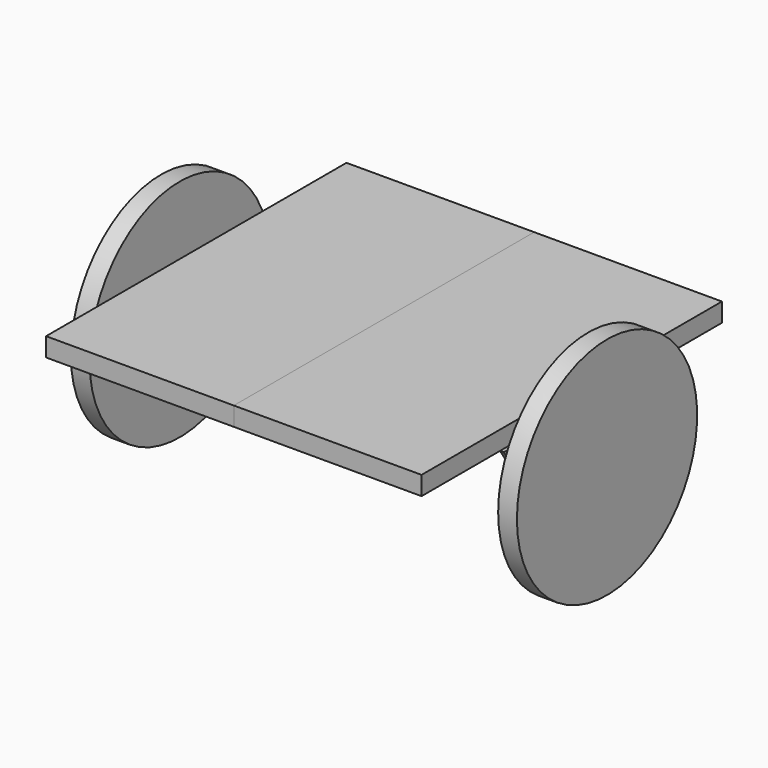
from build123d import *

# Parameters (mm, degrees)
F0_W      = 127
F0_H      = 254
F1_DEPTH  = 12.7
F3_DEPTH  = 11.176
F4_R      = 76.2
F5_DEPTH  = 12.7
F7_DEPTH  = 2.54
F12_R     = 6.556935049
F13_DEPTH = 12.7
F14_W     = 20.32
F14_H     = 45.72
F15_DEPTH = 6.35
F16_W     = 20.32
F16_H     = 22.86
F17_DEPTH = 29.972
F19_START = -3.81
F18_R     = 26.2593452301
F19_DEPTH = 11.43


# Not quite as in the source:
# - a feature names something its author has since deleted; it is built from what else it names
# - the program builds the solid bodies; features that only make, move or delete a surface that nothing else refers to are left out


with BuildPart() as f1:
    # F0 (on Top) → F1 (new body)
    with BuildSketch(Plane.XY):
        with Locations((-18.5930197371, 35.8398522526)):
            Rectangle(F0_W, F0_H)
    extrude(amount=F1_DEPTH)


with BuildPart() as f3:
    # F2 (on face) → F3 (new body)
    with BuildSketch(Plane(origin=(-82.0930197371, 0, 0), x_dir=(0, -1, 0), z_dir=(-1, 0, 0))):
        with BuildLine():
            ThreePointArc((-35.8398522526, -20.2696001321), (-40.3299803131, -31.1097281926), (-29.4898522526, -26.6196001321))
            ThreePointArc((-29.4898522526, -26.6196001321), (-31.3497241921, -22.1294720716), (-35.8398522526, -20.2696001321))
        make_face()
    extrude(amount=F3_DEPTH)

    # F4 (on face) → F5 (join)
    with BuildSketch(Plane(origin=(-93.2690197371, 0, 0), x_dir=(0, -1, 0), z_dir=(-1, 0, 0))):
        with Locations((-35.8398522526, -26.6196001321)):
            Circle(F4_R)
    extrude(amount=F5_DEPTH)

    # F6 (on face) → F7 (join)
    with BuildSketch(Plane(origin=(-82.0930197371, 0, 0), x_dir=(0, -1, 0), z_dir=(-1, 0, 0))):
        Polygon((0, 0), (-35.8398522526, 0), (-35.8398522526, -38.0577035248), (-35.8398522526, -38.1214432418), (0, -38.1214432418), (24.76891689, 0), align=None)
        Polygon((-35.8398522526, -38.0577035248), (-35.8398522526, 0), (-77.4306133389, 0), (-105.3093969822, 0), (-77.4306133389, -38.0577035248), align=None)
    extrude(amount=F7_DEPTH)


with BuildPart() as f11_1:
    # F11: instance of F3
    add(f3.part.mirror(Plane.YZ.offset(44.9069802629)))


with BuildPart() as f11_2:
    # F11: instance of F1
    add(f1.part.mirror(Plane.YZ.offset(44.9069802629)))


with BuildPart() as f13:
    # F12 (on face) → F13 (new body)
    with BuildSketch(Plane(origin=(0, 0, 0), x_dir=(1, 0, 0), z_dir=(0, 0, -1))):
        with Locations((44.9069802629, -137.7687752247)):
            Circle(F12_R)
    extrude(amount=F13_DEPTH)

    # F14 (on face) → F15 (join)
    with BuildSketch(Plane(origin=(0, 0, -12.7), x_dir=(1, 0, 0), z_dir=(0, 0, -1))):
        with Locations((45.2361442149, -135.3118325615)):
            Rectangle(F14_W, F14_H)
    extrude(amount=F15_DEPTH)

    # F16 (on face) → F17 (join)
    with BuildSketch(Plane(origin=(0, 0, -19.05), x_dir=(1, 0, 0), z_dir=(0, 0, -1))):
        with Locations((45.2361442149, -146.7418325615)):
            Rectangle(F16_W, F16_H)
    extrude(amount=F17_DEPTH)

    # F18 (on face) → F19 (join)
    with BuildSketch(Plane.YZ.offset(55.3961442149).offset(F19_START)):
        with Locations((146.7418325615, -49.022)):
            Circle(F18_R)
    extrude(amount=-F19_DEPTH)


solid = Compound([f1.part, f3.part, f11_1.part, f11_2.part, f13.part])
